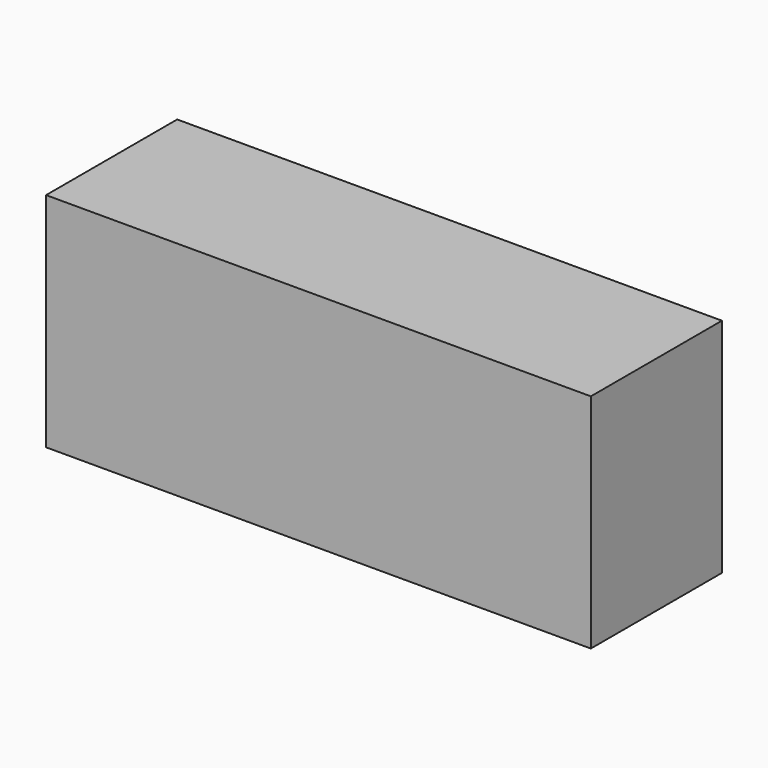
from build123d import *

# Parameters (mm, degrees)
F0_W     = 84.4493508339
F0_H     = 34.4211012125
F1_DEPTH = 25.4


# Not quite as in the source:
# - a feature of the source that left no trace in its solid (it failed there, or was rolled back) is left out


with BuildPart() as f1:
    # F0 (on Front) → F1 (new body)
    with BuildSketch(Plane.XZ):
        with Locations((6.6744517535, -2.4817334488)):
            Rectangle(F0_W, F0_H)
    extrude(amount=F1_DEPTH)


solid = f1.part
